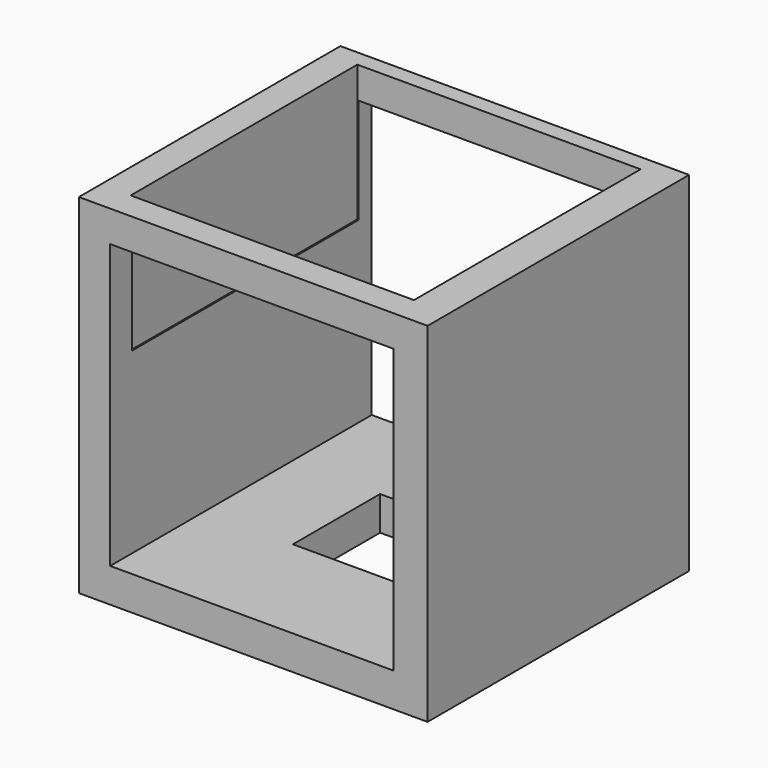
from build123d import *

# Parameters (mm, degrees)
F0_W     = 32
F0_H     = 32
F1_DEPTH = 30
F2_W     = 26
F2_H     = 26
F3_DEPTH = 30.001
F4_W     = 26
F4_H     = 26
F5_DEPTH = 12.5
F6_W     = 10
F6_H     = 10
F7_DEPTH = 32.001


# Not quite as in the source:
# - a feature names something its author has since deleted; it is built from what else it names


with BuildPart() as f1:
    # F0 (on Front) → F1 (new body)
    with BuildSketch(Plane.XZ):
        with Locations((-32.1818544654, 23.1859142184)):
            Rectangle(F0_W, F0_H)
    extrude(amount=F1_DEPTH)

    # F2 (on Front) → F3 (cut, through all)
    with BuildSketch(Plane.XZ):
        with Locations((-32.3113440342, 23.315487102)):
            Rectangle(F2_W, F2_H)
    extrude(amount=F3_DEPTH, mode=Mode.SUBTRACT)

    # F4 (on face) → F5 (cut, symmetric)
    with BuildSketch(Plane.XY.offset(39.1859142184)):
        with Locations((-32.4389154911, -14.4897329509)):
            Rectangle(F4_W, F4_H)
    extrude(amount=F5_DEPTH, both=True, mode=Mode.SUBTRACT)

    # F6 (on face) → F7 (cut, through all)
    with BuildSketch(Plane(origin=(0, 0, 7.1859142184), x_dir=(1, 0, 0), z_dir=(0, 0, -1))):
        with Locations((-32.1818544654, 14.1996787861)):
            Rectangle(F6_W, F6_H)
    extrude(amount=-F7_DEPTH, mode=Mode.SUBTRACT)


solid = f1.part
